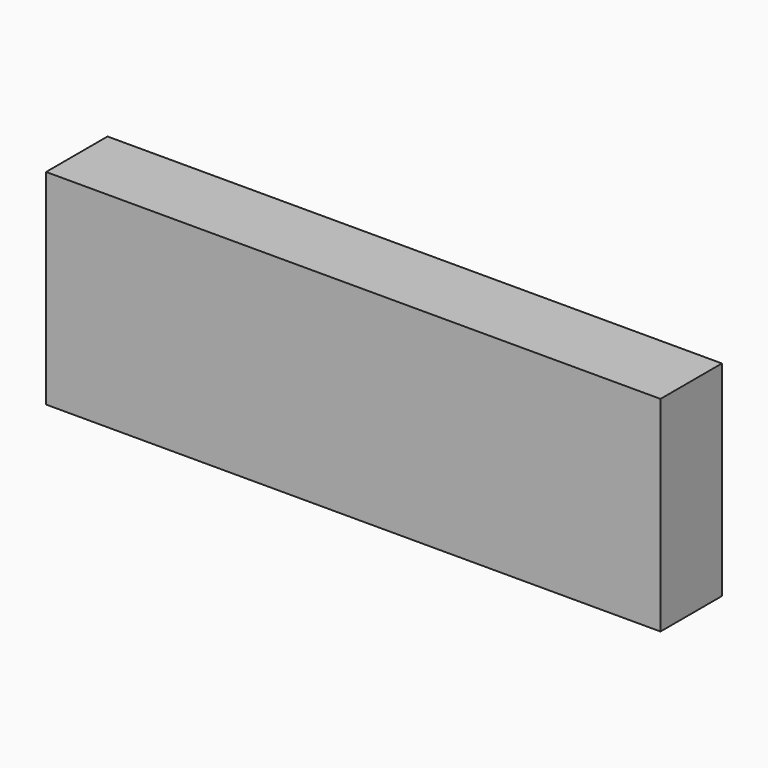
from build123d import *

# Parameters (mm, degrees)
F1_W     = 152.4
F1_H     = 50.8
F2_DEPTH = 9.525


# Not quite as in the source:
# - a variable given as a bare number and used for a length is read in inches; the dataset says mm whatever the document's units were


with BuildPart() as f2:
    # F1 (on Front) → F2 (new body, symmetric)
    with BuildSketch(Plane.XZ):
        Rectangle(F1_W, F1_H)
    extrude(amount=F2_DEPTH, both=True)


solid = f2.part
